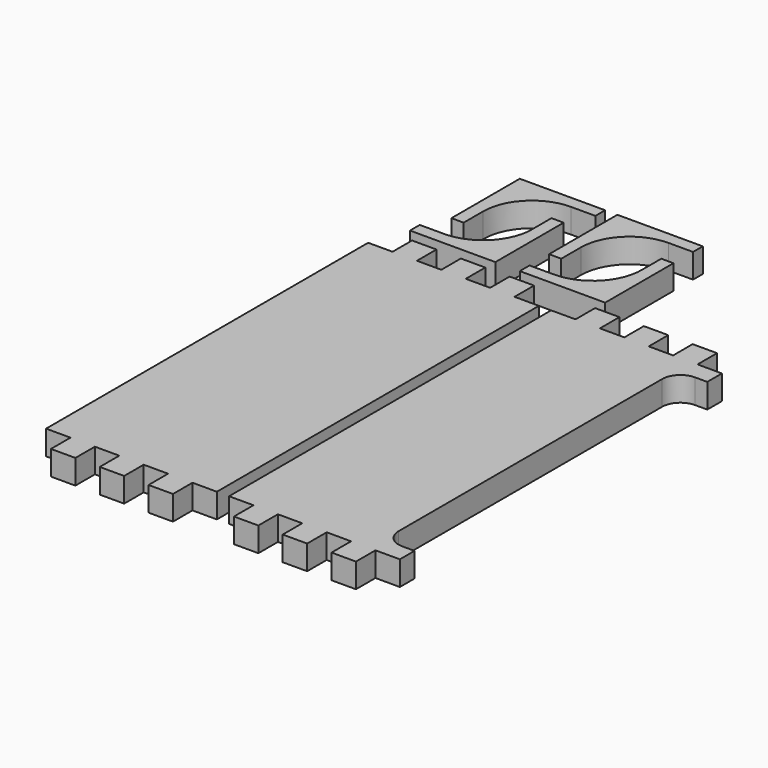
from build123d import *

# Parameters (mm, degrees)
F1_DEPTH  = 20
F4_W      = 150
F4_H      = 20
F5_DEPTH  = 25
F6_R      = 15
F8_DEPTH  = 20
F9_R      = 40
F11_ANGLE = 180


# Not quite as in the source:
# - a feature names something its author has since deleted; it is built from what else it names


with BuildPart() as f1:
    # F0 (on Top) → F1 (new body)
    with BuildSketch(Plane.XY):
        Polygon((-70, 190), (-70, 25), (-50, 25), (-50, 5), (-30, 5), (-30, 25), (-10, 25), (-10, 5), (10, 5), (10, 25), (30, 25), (30, 5), (50, 5), (50, 25), (70, 25), (70, 190), (70, 355), (50, 355), (50, 375), (30, 375), (30, 355), (10, 355), (10, 375), (-10, 375), (-10, 355), (-30, 355), (-30, 375), (-50, 375), (-50, 355), (-70, 355), align=None)
    extrude(amount=F1_DEPTH)


with BuildPart() as f2_1:
    # F2: copy of F1
    add(f1.part)


with BuildPart() as f2_1_1:
    # F3: moved
    add(f2_1.part.moved(Location((150, 0, 0))))

    # F4 (on face) → F5 (cut)
    with BuildSketch(Plane.YZ.offset(220)):
        with Locations((115, 10)):
            Rectangle(F4_W, F4_H)
        with Locations((265, 10)):
            Rectangle(F4_W, F4_H)
    extrude(amount=-F5_DEPTH, mode=Mode.SUBTRACT)

    # F6
    f6_edges = [f2_1_1.edges().sort_by_distance(p)[0] for p in [
        (195, 40, 10),
        (195, 340, 10),
    ]]
    fillet(f6_edges, radius=F6_R)


with BuildPart() as f8:
    # F7 (on face) → F8 (new body)
    with BuildSketch(Plane.XY.offset(20)):
        Polygon((-49.658793956, 484.9348437786), (-49.658793956, 414.9348437786), (-39.658793956, 414.9348437786), (-39.658793956, 474.9348437786), (20.341206044, 474.9348437786), (20.341206044, 484.9348437786), align=None)
    extrude(amount=-F8_DEPTH)

    # F9
    f9_edges = [f8.edges().sort_by_distance(p)[0] for p in [
        (-39.658794, 474.934844, 10),
    ]]
    fillet(f9_edges, radius=F9_R)


with BuildPart() as f10_1:
    # F10: copy of F8
    add(f8.part.moved(Location((80, 0, 0))))


with BuildPart() as f11_1:
    # F11: copy of F8
    add(f8.part.rotate(Axis((-49.658793956, 484.9348437786, 10), (0, 0, 1)), F11_ANGLE))


with BuildPart() as f12_1:
    # F12: copy of F11_1
    add(f11_1.part.moved(Location((60, -100, 0))))


with BuildPart() as f11_1_1:
    # F13: moved
    add(f11_1.part.moved(Location((150, -100, 0))))


solid = Compound([f1.part, f2_1_1.part, f8.part, f10_1.part, f12_1.part, f11_1_1.part])
